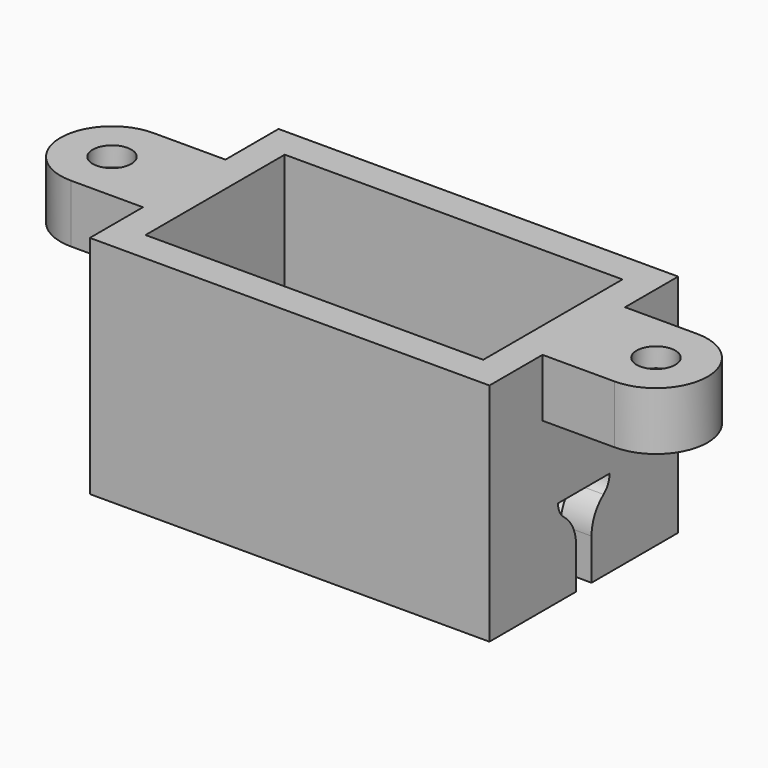
from build123d import *

# Parameters (mm, degrees)
F0_W      = 31
F0_H      = 18.3
F0_W_2    = 26.2
F0_H_2    = 13.5
F1_DEPTH  = 17.5
F2_W      = 26.2
F2_H      = 13.5
F2_W_2    = 22.2
F2_H_2    = 9.5
F3_DEPTH  = 2
F4_SIZE   = 1.99999
F6_START  = 13
F5_R      = 1.5
F6_DEPTH  = 4.5
F8_DEPTH  = 3
F10_DEPTH = 5
F11_R     = 1.49999
F12_R     = 3


# Not quite as in the source:
# - a fillet or chamfer is up to 0.001 mm smaller than in the source, because OpenCascade refuses the exact size


with BuildPart() as f1:
    # F0 (on Top) → F1 (new body)
    with BuildSketch(Plane.XY):
        Rectangle(F0_W, F0_H)
        Rectangle(F0_W_2, F0_H_2, mode=Mode.SUBTRACT)
    extrude(amount=F1_DEPTH)

    # F2 (on face) → F3 (join)
    with BuildSketch(Plane(origin=(0, 0, 0), x_dir=(1, 0, 0), z_dir=(0, 0, -1))):
        Rectangle(F2_W, F2_H)
        Rectangle(F2_W_2, F2_H_2, mode=Mode.SUBTRACT)
    extrude(amount=-F3_DEPTH)

    # F4 (size 2 in the source; OpenCascade refuses exactly that, so slightly less here)
    f4_edges = [f1.edges().sort_by_distance(p)[0] for p in [
        (0, 4.75, 2),
        (11.1, 0, 2),
        (0, -4.75, 2),
        (-11.1, 0, 2),
    ]]
    chamfer(f4_edges, length=F4_SIZE)

    # F5 (on Top) → F6 (join)
    with BuildSketch(Plane.XY.offset(F6_START)):
        with BuildLine():
            Line((17.1, -4), (21.1, -4))
            ThreePointArc((21.1, -4), (25.1, 0), (21.1, 4))
            Line((21.1, 4), (17.1, 4))
            Line((17.1, 4), (15.5, 4))
            Line((15.5, 4), (15.5, -4))
            Line((15.5, -4), (17.1, -4))
        make_face()
        with Locations((21.1, 0)):
            Circle(F5_R, mode=Mode.SUBTRACT)
        with BuildLine():
            ThreePointArc((-21.1, 4), (-25.1, 0), (-21.1, -4))
            Line((-21.1, -4), (-17.1, -4))
            Line((-17.1, -4), (-15.5, -4))
            Line((-15.5, -4), (-15.5, 4))
            Line((-15.5, 4), (-17.1, 4))
            Line((-17.1, 4), (-21.1, 4))
        make_face()
        with Locations((-21.1, 0)):
            Circle(F5_R, mode=Mode.SUBTRACT)
    extrude(amount=F6_DEPTH)

    # F7 (on face) → F8 (cut)
    with BuildSketch(Plane(origin=(0, 0, 13), x_dir=(1, 0, 0), z_dir=(0, 0, -1))):
        Polygon((22.6877132403, 2.75), (19.5122867597, 2.75), (17.9245735195, 0), (19.5122867597, -2.75), (22.6877132403, -2.75), (24.2754264805, 0), align=None)
        Polygon((-19.5122867597, 2.75), (-22.6877132403, 2.75), (-24.2754264805, 0), (-22.6877132403, -2.75), (-19.5122867597, -2.75), (-17.9245735195, 0), align=None)
    extrude(amount=-F8_DEPTH, mode=Mode.SUBTRACT)

    # F9 (on face) → F10 (cut)
    with BuildSketch(Plane.YZ.offset(15.5)):
        Polygon((0.75, 5.25), (2.5, 5.25), (2.5, 6.75), (-2.5, 6.75), (-2.5, 5.25), (-0.75, 5.25), (-0.75, 0), (0.75, 0), align=None)
    extrude(amount=-F10_DEPTH, mode=Mode.SUBTRACT)

    # F11 (radius 1.5 in the source; OpenCascade refuses exactly that, so slightly less here)
    f11_edges = [f1.edges().sort_by_distance(p)[0] for p in [
        (14.3, -2.5, 5.25),
        (14.3, 2.5, 5.25),
    ]]
    fillet(f11_edges, radius=F11_R)

    # F12
    f12_edges = [f1.edges().sort_by_distance(p)[0] for p in [
        (14.3, -0.75, 5.25),
        (14.3, 0.75, 5.25),
    ]]
    fillet(f12_edges, radius=F12_R)


solid = f1.part
